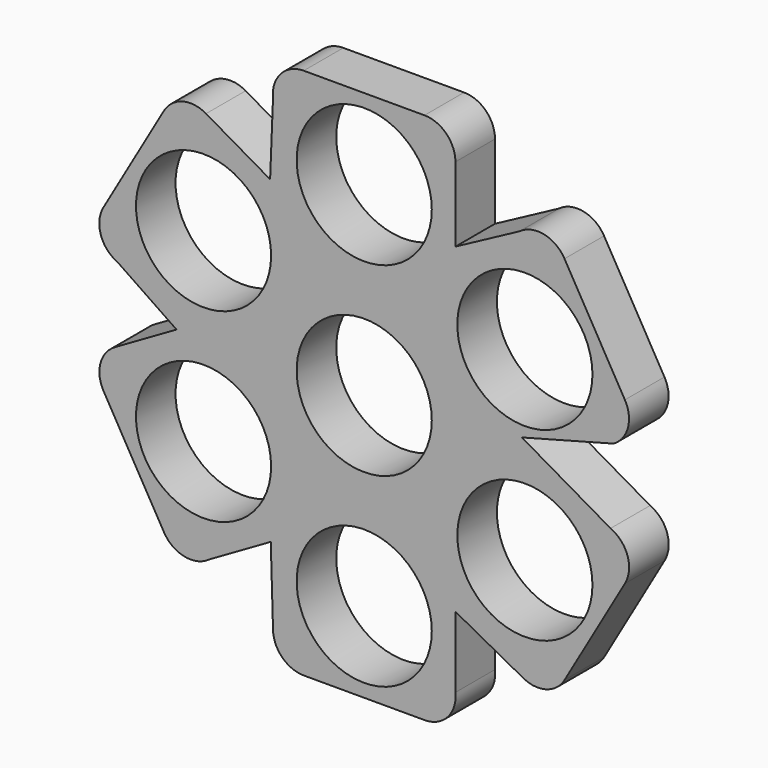
from build123d import *

# Parameters (mm, degrees)
F0_R     = 10.925
F1_DEPTH = 8


# Not quite as in the source:
# - a feature names something its author has since deleted; it is built from what else it names


with BuildPart() as f1:
    # F0 (on Front) → F1 (new body)
    with BuildSketch(Plane.XZ):
        with BuildLine():
            ThreePointArc((-164.4608943756, 109.2849649489), (-165.9253604697, 112.8204988548), (-169.4608943756, 114.2849649489))
            Line((-169.4608943756, 114.2849649489), (-188.9884267566, 114.2849649489))
            ThreePointArc((-188.9884267566, 114.2849649489), (-192.7173858315, 112.6158603567), (-193.95673582, 108.7229106361))
            Line((-193.95673582, 108.7229106361), (-194.4236024673, 97.0532244981))
            Line((-194.4236024673, 97.0532244981), (-204.7831671065, 103.0343219313))
            ThreePointArc((-204.7831671065, 103.0343219313), (-208.577262332, 103.5338240438), (-211.6132941254, 101.2041949124))
            Line((-211.6132941254, 101.2041949123), (-221.3770596376, 84.2928569721))
            ThreePointArc((-221.3770596376, 84.2928569721), (-221.7960530872, 80.2289308569), (-219.0443345156, 77.209146778))
            Line((-219.0443345156, 77.209146778), (-209.5551351868, 70.7485068424))
            Line((-209.5551351868, 70.7485068424), (-219.5310878287, 64.9888878992))
            ThreePointArc((-219.5310878287, 64.9888878992), (-221.8607169602, 61.9528561057), (-221.3612148477, 58.1587608802))
            Line((-221.3612148477, 58.1587608802), (-211.5974493355, 41.24742294))
            ThreePointArc((-211.5974493355, 41.24742294), (-208.2874828054, 38.852600911), (-204.2964137934, 39.7257670587))
            Line((-204.2964137934, 39.7257670587), (-194.3204611514, 45.4853860019))
            Line((-194.3204611514, 45.4853860019), (-193.95673582, 33.1940968847))
            ThreePointArc((-193.95673582, 33.1940968847), (-192.492269726, 29.6585629787), (-188.95673582, 28.1940968847))
            Line((-188.95673582, 28.1940968847), (-169.4292047957, 28.1940968847))
            ThreePointArc((-169.4292047957, 28.1940968847), (-165.7002448161, 29.8632009709), (-164.4608943756, 33.7561511974))
            Line((-164.4608943756, 33.7561511974), (-164.4608943756, 45.2587688032))
            Line((-164.4608943756, 45.2587688032), (-153.6344630891, 39.4447399023))
            ThreePointArc((-153.6344630891, 39.4447399023), (-149.8403678636, 38.9452377897), (-146.8043360702, 41.2748669212))
            Line((-146.8043360702, 41.2748669212), (-137.040570558, 58.1862048614))
            ThreePointArc((-137.040570558, 58.1862048614), (-136.6215771084, 62.2501309766), (-139.37329568, 65.2699150555))
            Line((-139.37329568, 65.2699150555), (-153.7136262629, 73.5493087778))
            Line((-153.7136262629, 73.5493087778), (-138.8865423669, 77.4901739344))
            ThreePointArc((-138.8865423669, 77.4901739344), (-136.5569132354, 80.5262057278), (-137.056415348, 84.3203009533))
            Line((-137.056415348, 84.3203009533), (-146.8201808601, 101.2316388936))
            ThreePointArc((-146.8201808601, 101.2316388936), (-150.1301473902, 103.6264609225), (-154.1212164023, 102.7532947749))
            Line((-154.1212164023, 102.7532947749), (-164.4608943756, 97.2202930303))
            Line((-164.4608943756, 97.2202930303), (-164.4608943756, 109.2849649489))
        make_face()
        with Locations((-179.2088150978, 41.2395309168)):
            Circle(F0_R, mode=Mode.SUBTRACT)
        with Locations((-205.1895772113, 56.2395309168)):
            Circle(F0_R, mode=Mode.SUBTRACT)
        with Locations((-153.2280529843, 56.2395309168)):
            Circle(F0_R, mode=Mode.SUBTRACT)
        with Locations((-205.1895772113, 86.2395309168)):
            Circle(F0_R, mode=Mode.SUBTRACT)
        with Locations((-179.2088150978, 71.2395309168)):
            Circle(F0_R, mode=Mode.SUBTRACT)
        with Locations((-179.2088150978, 101.2395309168)):
            Circle(F0_R, mode=Mode.SUBTRACT)
        with Locations((-153.2280529843, 86.2395309168)):
            Circle(F0_R, mode=Mode.SUBTRACT)
    extrude(amount=F1_DEPTH)


solid = f1.part
